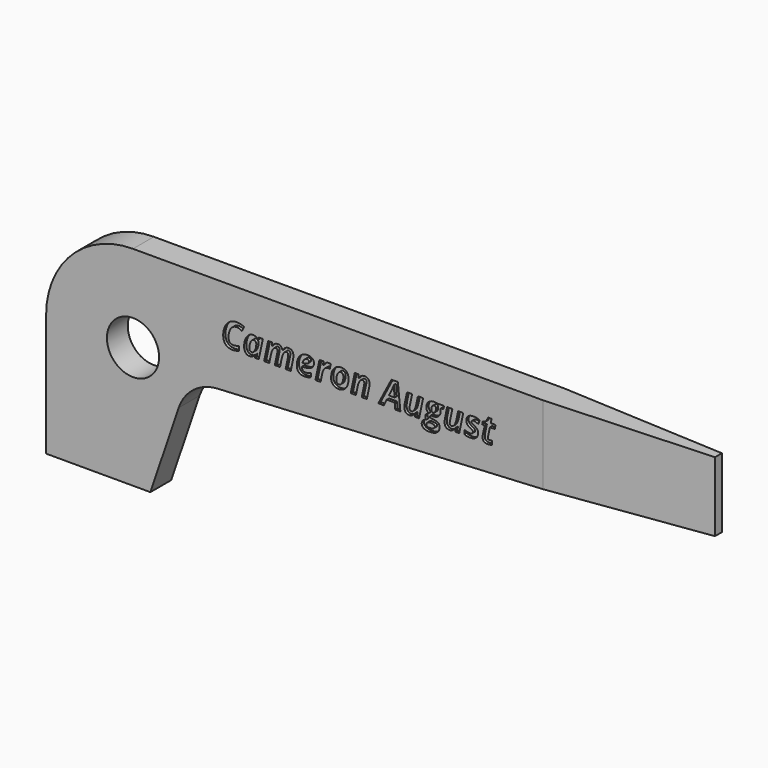
from build123d import *

# Parameters (mm, degrees)
F1_DEPTH     = 2.38125
F2_R         = 2.38125
F3_DEPTH     = 2.38225
F5_DEPTH     = 19.051
F6_TEXT_SIZE = 3.2069937636
F7_DEPTH     = 0.254


# Not quite as in the source:
# - Text() gives the source's letters only with a copy of the font that has no kerning and outlines rounded to 1/6400 em; it was checked with that copy


with BuildPart() as f1:
    # F0 (on Front) → F1 (new body)
    with BuildSketch(Plane.XZ):
        with BuildLine():
            Line((60.4544878006, 19.05), (7.9375, 19.05))
            ThreePointArc((7.9375, 19.05), (2.3248399243, 16.7251600757), (0, 11.1125))
            Line((0, 11.1125), (0, 0))
            Line((0, 0), (9.525, 0))
            Line((9.525, 0), (12.1103451907, 7.6262422093))
            ThreePointArc((12.1103451907, 7.6262422093), (13.4739996894, 9.5180621078), (15.6640309888, 10.3194977121))
            Line((15.6640309888, 10.3194977121), (60.4544878006, 12.7))
            Line((60.4544878006, 12.7), (60.4544878006, 19.05))
        make_face()
    extrude(amount=F1_DEPTH)

    # F2 (on face) → F3 (cut, through all)
    with BuildSketch(Plane.XZ.offset(2.38125)):
        with Locations((7.9375, 11.1125)):
            Circle(F2_R)
    extrude(amount=-F3_DEPTH, mode=Mode.SUBTRACT)

    # F4 (on face) → F5 (cut, through all)
    with BuildSketch(Plane.XY.offset(19.05)):
        Polygon((60.4544878006, 0), (45.3732378006, 0), (60.4544878006, -0.79375), align=None)
        Polygon((60.4544878006, -2.38125), (60.4544878006, -1.5875), (45.3732378006, -2.38125), align=None)
    extrude(amount=-F5_DEPTH, mode=Mode.SUBTRACT)

    # F6 (on face) → F7 (cut)
    with BuildSketch(Plane.XZ.offset(2.38125)):
        with Locations((15.9833636135, 13.9114577323)):
            Text('Cameron August', F6_TEXT_SIZE, font='Open Sans', font_style=FontStyle.BOLDITALIC, text_align=(TextAlign.LEFT, TextAlign.BOTTOM))
    extrude(amount=-F7_DEPTH, mode=Mode.SUBTRACT)


solid = f1.part
